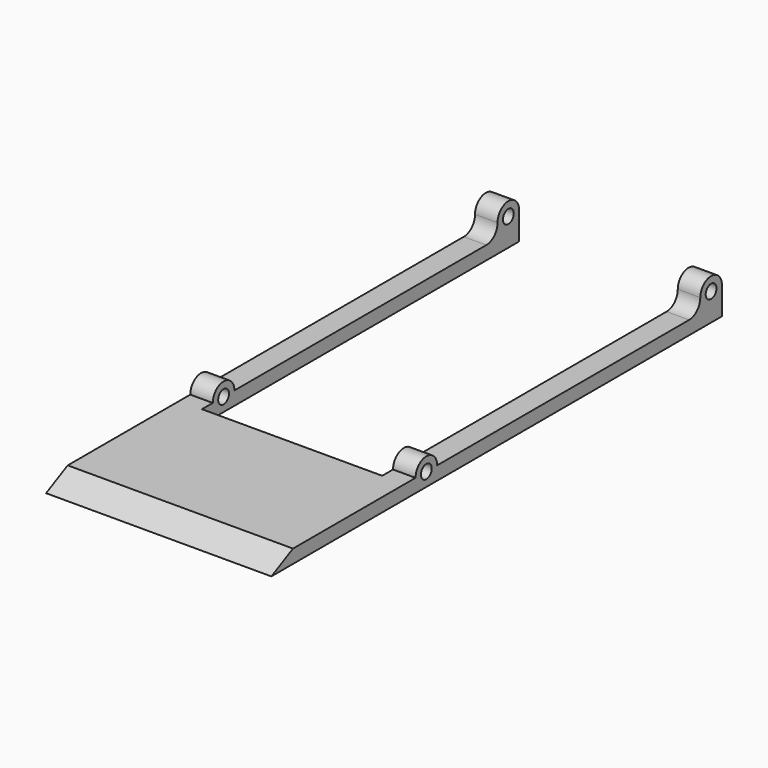
from build123d import *

# Parameters (mm, degrees)
F1_DEPTH  = 3
F3_DEPTH  = 5
F5_DEPTH  = 5
F7_DEPTH  = 5
F9_DEPTH  = 5
F11_R     = 1.5
F12_DEPTH = 55
F14_DEPTH = 100


# Not quite as in the source:
# - a pattern or mirror of a feature is missing from the dataset's text; its kind, count and spacing are read off the source's solid
# - a feature names something its author has since deleted; it is built from what else it names


with BuildPart() as f1:
    # F0 (on Top) → F1 (new body)
    with BuildSketch(Plane.XY):
        Polygon((-20, 62.5), (-25, 62.5), (-25, -62.5), (25, -62.5), (25, 62.5), (20, 62.5), (20, -25.5), (-20, -25.5), align=None)
    extrude(amount=F1_DEPTH)

    # F4 (on face) → F5 (join)
    with BuildSketch(Plane(origin=(-25, 0, 0), x_dir=(0, -1, 0), z_dir=(-1, 0, 0))):
        with BuildLine():
            Line((16.5, 3), (22.5, 3))
            ThreePointArc((22.5, 3), (19.5, 6), (16.5, 3))
        make_face()
    f5 = extrude(amount=-F5_DEPTH)

    # F5_copies: F5 across plane
    add(f5.mirror(Plane(origin=(0, 0, 0), x_dir=(0, 0, 1), z_dir=(1, 0, 0))))

    # F6 (on face) → F7 (join)
    with BuildSketch(Plane(origin=(-25, 0, 0), x_dir=(0, -1, 0), z_dir=(-1, 0, 0))):
        with BuildLine():
            Line((-62.5, 6.1), (-62.5, 3))
            Line((-62.5, 3), (-56.5, 3))
            Line((-56.5, 3), (-56.5, 6.1))
            ThreePointArc((-56.5, 6.1), (-59.5, 3.1), (-62.5, 6.1))
        make_face()
        with BuildLine():
            ThreePointArc((-56.5, 6.1), (-59.5, 9.1), (-62.5, 6.1))
            Line((-62.5, 6.1), (-61, 6.1))
            ThreePointArc((-61, 6.1), (-59.5, 7.6), (-58, 6.1))
            Line((-58, 6.1), (-56.5, 6.1))
        make_face()
        with BuildLine():
            Line((-56.5, 6.1), (-56.5, 3))
            Line((-56.5, 3), (-53.4, 3))
            ThreePointArc((-53.4, 3), (-55.5920310217, 3.9079689783), (-56.5, 6.1))
        make_face()
        with BuildLine():
            Line((-61, 6.1), (-62.5, 6.1))
            ThreePointArc((-62.5, 6.1), (-59.5, 3.1), (-56.5, 6.1))
            Line((-56.5, 6.1), (-58, 6.1))
            ThreePointArc((-58, 6.1), (-59.5, 4.6), (-61, 6.1))
        make_face()
    extrude(amount=-F7_DEPTH)

    # F8 (on face) → F9 (join)
    with BuildSketch(Plane.YZ.offset(25)):
        with BuildLine():
            Line((61, 6.1), (62.5, 6.1))
            ThreePointArc((62.5, 6.1), (59.5, 9.1), (56.5, 6.1))
            Line((56.5, 6.1), (58, 6.1))
            ThreePointArc((58, 6.1), (59.5, 7.6), (61, 6.1))
        make_face()
        with BuildLine():
            Line((56.5, 3), (62.5, 3))
            Line((62.5, 3), (62.5, 6.1))
            ThreePointArc((62.5, 6.1), (59.5, 3.1), (56.5, 6.1))
            Line((56.5, 6.1), (56.5, 3))
        make_face()
        with BuildLine():
            Line((53.4, 3), (56.5, 3))
            Line((56.5, 3), (56.5, 6.1))
            ThreePointArc((56.5, 6.1), (55.5920310217, 3.9079689783), (53.4, 3))
        make_face()
        with BuildLine():
            ThreePointArc((56.5, 6.1), (59.5, 3.1), (62.5, 6.1))
            Line((62.5, 6.1), (61, 6.1))
            ThreePointArc((61, 6.1), (59.5, 4.6), (58, 6.1))
            Line((58, 6.1), (56.5, 6.1))
        make_face()
    extrude(amount=-F9_DEPTH)


with BuildPart() as f3:
    # F2 (on face) → F3 (new body)
    with BuildSketch(Plane.YZ.offset(25)):
        with BuildLine():
            ThreePointArc((-19.5000000146, 0), (-17.3786796616, 0.8786796513), (-16.5, 3))
            Line((-16.5, 3), (-22.5, 3))
            ThreePointArc((-22.5, 3), (-21.6213203487, 0.8786796616), (-19.5000000146, 0))
        make_face()
    extrude(amount=-F3_DEPTH)


with BuildPart() as f1_1:
    add(f1.part)

    # F10: union F3
    add(f3.part)

    # F11 (on face) → F12 (cut)
    with BuildSketch(Plane.YZ.offset(25)):
        with Locations((-19.5, 3)):
            Circle(F11_R)
    extrude(amount=-F12_DEPTH, mode=Mode.SUBTRACT)

    # F13 (on face) → F14 (cut)
    with BuildSketch(Plane.YZ.offset(25)):
        Polygon((-62.5, 3), (-62.5, 0), (-56.5, 3), align=None)
    extrude(amount=-F14_DEPTH, mode=Mode.SUBTRACT)


solid = f1_1.part
